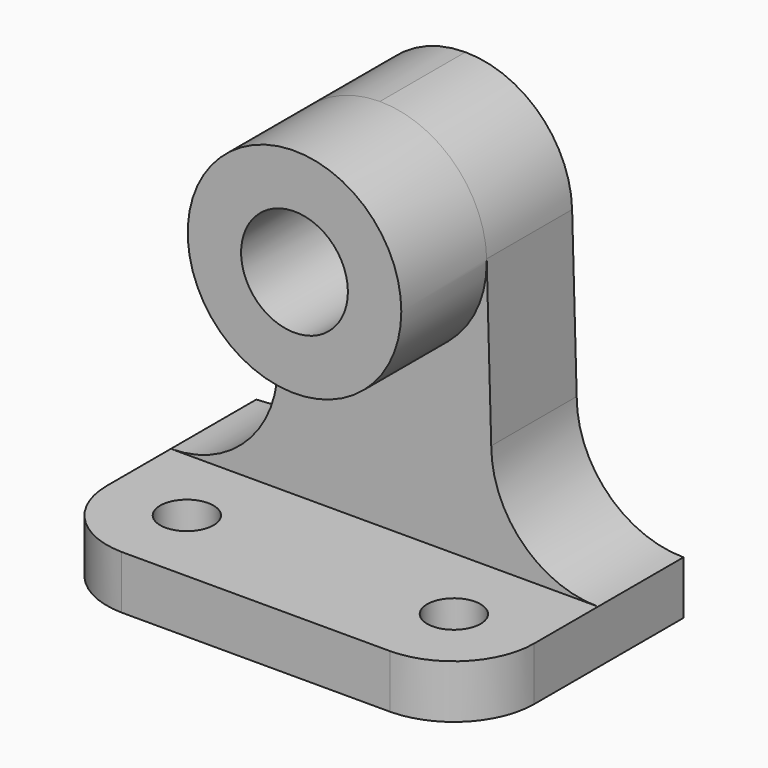
from build123d import *

# Parameters (mm, degrees)
F0_W      = 50.8
F0_H      = 31.75
F1_DEPTH  = 6.35
F2_W      = 50.8
F2_H      = 12.7
F3_DEPTH  = 44.45
F4_R      = 3.175
F5_DEPTH  = 6.35
F6_R      = 6.35
F7_DEPTH  = 12.7
F8_R      = 12.7
F9_DEPTH  = 12.7
F10_R     = 6.35
F11_DEPTH = 25.4


# Not quite as in the source:
# - after a boolean that leaves OpenCascade's solid faulty, fix() repairs it
# - a length typed as a fraction of an inch, garbled in the dataset ("3 / 203.2 mm" for 3/8 in), is restored


with BuildPart() as f1:
    # F0 (on Top) → F1 (new body)
    with BuildSketch(Plane.XY):
        with Locations((16.015455, 9.347902)):
            Rectangle(F0_W, F0_H)
    extrude(amount=F1_DEPTH)

    # F2 (on face) → F3 (join)
    with BuildSketch(Plane.XY.offset(6.35)):
        with Locations((16.015455, 18.872902)):
            Rectangle(F2_W, F2_H)
    extrude(amount=F3_DEPTH)

    # F4 (on face) → F5 (cut)
    with BuildSketch(Plane.XY.offset(6.35)):
        with Locations((0.140455, 2.997902)):
            Circle(F4_R)
        with Locations((31.890455, 2.997902)):
            Circle(F4_R)
        with BuildLine():
            ThreePointArc((41.415455, 2.997902), (38.618068, -3.729712), (31.890455, -6.527098))
            Line((31.890455, -6.527098), (41.415455, -6.527098))
            Line((41.415455, -6.527098), (41.415455, 2.997902))
        make_face()
        with BuildLine():
            ThreePointArc((0, -6.527098), (-6.63612, -3.679782), (-9.384545, 2.997902))
            Line((-9.384545, 2.997902), (-9.384545, -6.527098))
            Line((-9.384545, -6.527098), (0, -6.527098))
        make_face()
    extrude(amount=-F5_DEPTH, mode=Mode.SUBTRACT)

    # F6 (on face) → F7 (cut)
    with BuildSketch(Plane.XZ.offset(-12.522902)):
        with Locations((15.479321, 38.1)):
            Circle(F6_R)
        with BuildLine():
            Line((-9.384545, 50.8), (-9.384545, 19.05))
            Line((-9.384545, 19.05), (3.315455, 19.05))
            Line((3.315455, 19.05), (2.784444, 37.739306))
            ThreePointArc((2.784444, 37.739306), (6.372433, 46.951813), (15.479321, 50.8))
            Line((15.479321, 50.8), (-9.384545, 50.8))
        make_face()
        with BuildLine():
            Line((28.174386, 38.453994), (28.715455, 19.05))
            Line((28.715455, 19.05), (41.415455, 19.05))
            Line((41.415455, 19.05), (41.415455, 50.8))
            Line((41.415455, 50.8), (15.479321, 50.8))
            ThreePointArc((15.479321, 50.8), (24.333536, 47.204552), (28.174386, 38.453994))
        make_face()
        with BuildLine():
            Line((3.315455, 19.05), (-9.384545, 19.05))
            Line((-9.384545, 19.05), (-9.384545, 6.35))
            ThreePointArc((-9.384545, 6.35), (-0.404289, 10.069744), (3.315455, 19.05))
        make_face()
        with BuildLine():
            Line((41.415455, 19.05), (28.715455, 19.05))
            ThreePointArc((28.715455, 19.05), (32.435199, 10.069744), (41.415455, 6.35))
            Line((41.415455, 6.35), (41.415455, 19.05))
        make_face()
    extrude(amount=-F7_DEPTH, mode=Mode.SUBTRACT)

    # F8 (on face) → F9 (join)
    with BuildSketch(Plane.XZ.offset(-12.522902)):
        with Locations((15.479321, 38.1)):
            Circle(F8_R)
    extrude(amount=F9_DEPTH)

    add(f1.part.fix(), mode=Mode.REPLACE)

    # F10 (on face) → F11 (cut)
    with BuildSketch(Plane.XZ.offset(0.177098)):
        with Locations((15.479321, 38.1)):
            Circle(F10_R)
    extrude(amount=-F11_DEPTH, mode=Mode.SUBTRACT)


solid = f1.part
